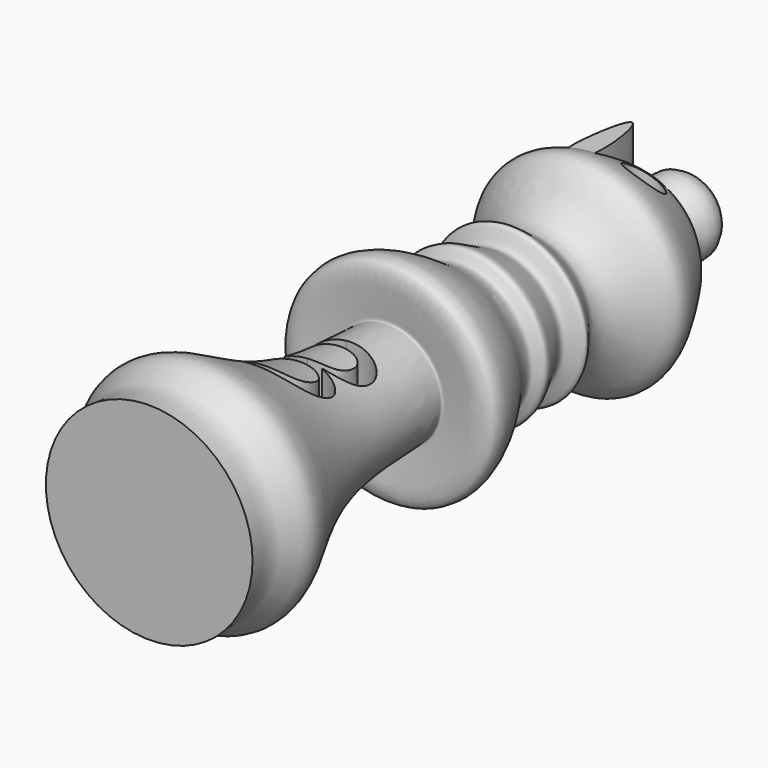
from build123d import *

# Parameters (mm, degrees)
F2_R          = 2.7566167547
F2_R_2        = 2.9848108926
F3_DEPTH      = 36.8
F3_DEPTH_BACK = 44.2
F4_TEXT_SIZE  = 26.4616941826
F5_DEPTH      = 64.5
F7_DEPTH      = 15.3


# Not quite as in the source:
# - Text() gives the source's letters only with a copy of the font that has no kerning and outlines rounded to 1/6400 em; it was checked with that copy


with BuildPart() as f1:
    # F0 (on Top) → F1 (revolve)
    with BuildSketch(Plane.XY):
        with BuildLine():
            Line((-40.0285758078, 58.5421025753), (-40.0285758078, 58.3114363253))
            Line((-40.0285758078, 58.3114363253), (-40.0285758078, -49.8705357313))
            Line((-40.0285758078, -49.8705357313), (-23.8820128143, -49.8705357313))
            add(Edge.make_bspline(
                [(-23.8820128143, -49.8705357313), (-24.1366999614, -48.2777367469), (-24.646866369, -45.0871849464), (-20.5693508763, -41.0534794981), (-24.2604169939, -34.1559647373), (-31.7267300587, -20.3577000414), (-31.5124490907, -4.2206512055), (-32.0012459265, -2.4376961198), (-19.9866080801, -5.9566241137), (-26.3517454808, 5.9784650645), (-28.0888253734, 7.6946354979), (-30.11467888, 11.6670061011), (-26.3138359258, 11.9206489504), (-30.7077434274, 17.6863496844), (-29.9459005165, 19.2683620092), (-26.1267685538, 20.0178765622), (-32.6980056031, 24.7646986893), (-27.7166995677, 30.2604139799), (-22.2520602764, 33.4908284532), (-26.5903192636, 40.5853060425), (-30.7164522984, 47.4178348756), (-38.2025191752, 48.0662583406), (-30.5345737871, 54.590846345), (-39.5231386773, 58.7014118858), (-40.0285758078, 58.5421025753)],
                knots=[0, 0, 0, 0, 0.041402215, 0.0829331968, 0.1323221314, 0.2122105524, 0.2875763081, 0.304039273, 0.3572213713, 0.4138100862, 0.4506224252, 0.4847653994, 0.5106380465, 0.5570010023, 0.5802831646, 0.6087183376, 0.6526048715, 0.7001901153, 0.7449210194, 0.7956984389, 0.8519187365, 0.8925218021, 0.9382066344, 0.9907421646, 0.9907421646, 0.9907421646, 0.9907421646], degree=3))
        make_face()
    revolve(axis=Axis((-40.0285758078, 2.6057958603, 0), (0, -1, 0)))

    # F2 (on Top) → F3 (cut, two sides)
    with BuildSketch(Plane.XY) as f3_sk:
        with Locations((-35.1398997009, 40.6340844929)):
            Circle(F2_R)
        with Locations((-48.4175160527, 40.6340844929)):
            Circle(F2_R_2)
    extrude(amount=F3_DEPTH, mode=Mode.SUBTRACT)
    extrude(f3_sk.sketch, amount=-F3_DEPTH_BACK, mode=Mode.SUBTRACT)

    # F4 (on Top) → F5 (cut)
    with BuildSketch(Plane.XY):
        with Locations((-48.9580482244, -29.0582366288)):
            Text('B', F4_TEXT_SIZE, font='Open Sans', text_align=(TextAlign.LEFT, TextAlign.BOTTOM))
    extrude(amount=F5_DEPTH, mode=Mode.SUBTRACT)

    # F6 (on Top) → F7 (join)
    with BuildSketch(Plane.XY):
        with BuildLine():
            add(Edge.make_bspline(
                [(-41.6431464255, 46.5423427522), (-42.6001240301, 46.8680742), (-44.0781250498, 37.7530815097), (-43.310820791, 34.5449514783), (-38.9073464817, 34.7382922887), (-40.5715572996, 46.1776003844), (-41.6431464255, 46.5423427522)],
                knots=[0, 0, 0, 0, 0.3055756523, 0.4976231006, 0.6578273676, 1, 1, 1, 1], degree=3))
        make_face()
    extrude(amount=F7_DEPTH)


solid = f1.part
